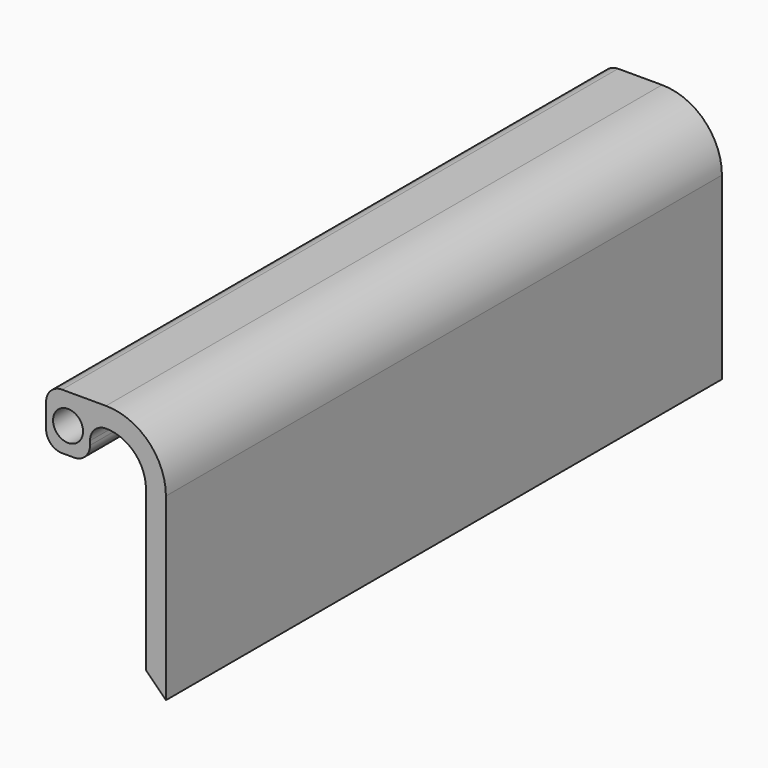
from build123d import *

# Parameters (mm, degrees)
F1_DEPTH = 17.4
F2_R     = 0.75
F3_DEPTH = 11
F4_R     = 0.79999
F5_SIZE  = 0.99999


# Not quite as in the source:
# - a fillet or chamfer is up to 0.001 mm smaller than in the source, because OpenCascade refuses the exact size
# - a pattern or mirror of a feature is missing from the dataset's text; its kind, count and spacing are read off the source's solid


with BuildPart() as f1:
    # F0 (on Front) → F1 (new body, symmetric)
    with BuildSketch(Plane.XZ):
        with BuildLine():
            ThreePointArc((3, -1), (4.4142135624, -1.5857864376), (5, -3))
            Line((5, -3), (5, -12))
            Line((5, -12), (6, -12))
            Line((6, -12), (6, -3))
            ThreePointArc((6, -3), (5.1213203436, -0.8786796564), (3, 0))
            Line((3, 0), (0, 0))
            Line((0, 0), (0, -2.8))
            Line((0, -2.8), (2.2, -2.8))
            Line((2.2, -2.8), (2.2, -1))
            Line((2.2, -1), (3, -1))
        make_face()
    extrude(amount=F1_DEPTH, both=True)

    # F2 (on face) → F3 (cut)
    with BuildSketch(Plane.XZ.offset(17.4)):
        with Locations((1.1, -1.5)):
            Circle(F2_R)
    f3 = extrude(amount=-F3_DEPTH, mode=Mode.SUBTRACT)

    # F3_copies: F3 across plane
    add(f3.mirror(Plane.ZX), mode=Mode.SUBTRACT)

    # F4 (radius 0.8 in the source; OpenCascade refuses exactly that, so slightly less here)
    f4_edges = [f1.edges().sort_by_distance(p)[0] for p in [
        (2.2, 0, -1),
        (2.2, 0, -2.8),
        (0, 0, -2.8),
        (0, 0, 0),
    ]]
    fillet(f4_edges, radius=F4_R)

    # F5 (size 1 in the source; OpenCascade refuses exactly that, so slightly less here)
    f5_edges = [f1.edges().sort_by_distance(p)[0] for p in [
        (5, 0, -12),
    ]]
    chamfer(f5_edges, length=F5_SIZE)


solid = f1.part
